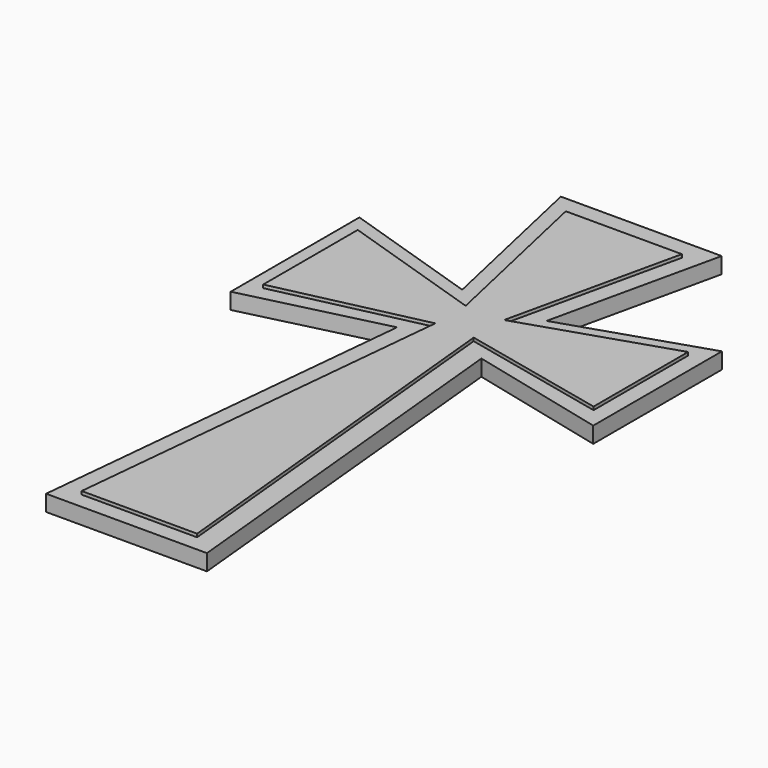
from build123d import *

# Parameters (mm, degrees)
F1_DEPTH = 5
F2_DEPTH = 6


# Not quite as in the source:
# - a feature names something its author has since deleted; it is built from what else it names


with BuildPart() as f1:
    # F0 (on Top) → F1 (new body)
    with BuildSketch(Plane.XY):
        Polygon((25, 78.4878924489), (0, 78.4878924489), (-25, 78.4878924489), (-13.1142183076, 25.3134854138), (-56.342728436, 39.404849359), (-56.342728436, -10.595150641), (-13.1142183076, 0), (-25, -121.5121075511), (0, -121.5121075511), (25, -121.5121075511), (13.1142183076, 0), (56.342728436, -10.595150641), (56.342728436, 39.404849359), (13.1142183076, 25.3134854138), align=None)
        Polygon((-18.0415231461, 71.7220325265), (0, 71.7220325265), (18.0415231461, 71.7220325265), (5.9721833782, 17.7264265097), (51.342728436, 32.5160378311), (51.342728436, -4.2216783711), (5.9721833782, 5.9197491293), (17.9479308986, -116.5121075511), (0, -116.5121075511), (-17.9479308986, -116.5121075511), (-5.9721833782, 5.9197491293), (-51.342728436, -4.2216783711), (-51.342728436, 32.5160378311), (-5.9721833782, 17.7264265097), align=None, mode=Mode.SUBTRACT)
        Polygon((18.0415231461, 71.7220325265), (0, 71.7220325265), (-18.0415231461, 71.7220325265), (-5.9721833782, 17.7264265097), (-51.342728436, 32.5160378311), (-51.342728436, -4.2216783711), (-5.9721833782, 5.9197491293), (-17.9479308986, -116.5121075511), (0, -116.5121075511), (17.9479308986, -116.5121075511), (5.9721833782, 5.9197491293), (51.342728436, -4.2216783711), (51.342728436, 32.5160378311), (5.9721833782, 17.7264265097), align=None)
    extrude(amount=F1_DEPTH)

    # F0 (on Top) → F2 (join)
    with BuildSketch(Plane.XY):
        Polygon((18.0415231461, 71.7220325265), (0, 71.7220325265), (-18.0415231461, 71.7220325265), (-5.9721833782, 17.7264265097), (-51.342728436, 32.5160378311), (-51.342728436, -4.2216783711), (-5.9721833782, 5.9197491293), (-17.9479308986, -116.5121075511), (0, -116.5121075511), (17.9479308986, -116.5121075511), (5.9721833782, 5.9197491293), (51.342728436, -4.2216783711), (51.342728436, 32.5160378311), (5.9721833782, 17.7264265097), align=None)
    extrude(amount=F2_DEPTH)


solid = f1.part
